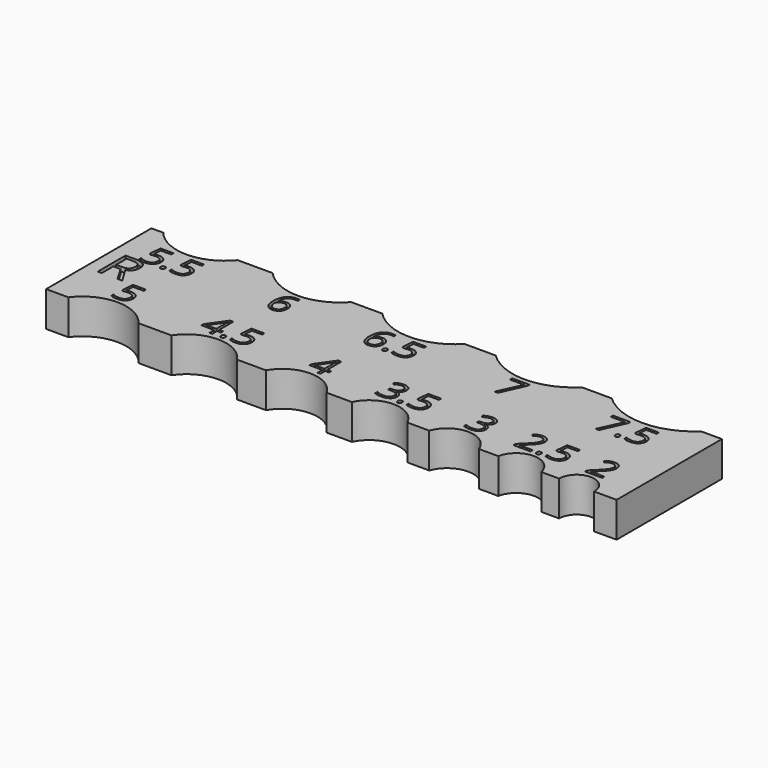
from build123d import *

# Parameters (mm, degrees)
F1_DEPTH       = 4
F2_TEXT_SIZE   = 4.1666666667
F2_TEXT_SIZE_2 = 5.5555555556
F3_DEPTH       = 0.5


# Not quite as in the source:
# - Text() gives the source's letters only with a copy of the font that has no kerning and outlines rounded to 1/6400 em; it was checked with that copy


with BuildPart() as f1:
    # F0 (on Top) → F1 (new body)
    with BuildSketch(Plane.XY):
        with BuildLine():
            Line((-84.5385417342, 32.5298000872), (-84.5385417342, 17.5298000872))
            Line((-84.5385417342, 17.5298000872), (-82.0045393762, 17.5298000872))
            ThreePointArc((-82.0045393762, 17.5298000872), (-78.0045393762, 19.5298000872), (-74.0045393762, 17.5298000872))
            Line((-74.0045393762, 17.5298000872), (-70.2570714699, 17.5298000872))
            ThreePointArc((-70.2570714699, 17.5298000872), (-66.5154140831, 19.5298000872), (-62.7737566964, 17.5298000872))
            Line((-62.7737566964, 17.5298000872), (-59.4914272166, 17.5298000872))
            ThreePointArc((-59.4914272166, 17.5298000872), (-56.0273256014, 19.5298000872), (-52.5632239863, 17.5298000872))
            Line((-52.5632239863, 17.5298000872), (-49.7027702811, 17.5298000872))
            ThreePointArc((-49.7027702811, 17.5298000872), (-46.5404926209, 19.5298000872), (-43.3782149608, 17.5298000872))
            Line((-43.3782149608, 17.5298000872), (-40.8836383714, 17.5298000872))
            ThreePointArc((-40.8836383714, 17.5298000872), (-38.0552112467, 19.5298000872), (-35.226784122, 17.5298000872))
            Line((-35.226784122, 17.5298000872), (-33.0213862159, 17.5298000872))
            ThreePointArc((-33.0213862159, 17.5298000872), (-30.5718964731, 19.5298000872), (-28.1224067304, 17.5298000872))
            Line((-28.1224067304, 17.5298000872), (-26.0911557747, 17.5298000872))
            ThreePointArc((-26.0911557747, 17.5298000872), (-24.0911557747, 19.5298000872), (-22.0911557747, 17.5298000872))
            Line((-22.0911557747, 17.5298000872), (-19.5385417342, 17.5298000872))
            Line((-19.5385417342, 17.5298000872), (-19.5385417342, 32.5298000872))
            Line((-19.5385417342, 32.5298000872), (-21.9044512947, 32.5298000872))
            ThreePointArc((-21.9044512947, 32.5298000872), (-27.0034708083, 30.5298000872), (-32.1024903219, 32.5298000872))
            Line((-32.1024903219, 32.5298000872), (-35.5119116897, 32.5298000872))
            ThreePointArc((-35.5119116897, 32.5298000872), (-40.4108911753, 30.5298000872), (-45.3098706608, 32.5298000872))
            Line((-45.3098706608, 32.5298000872), (-48.8570836346, 32.5298000872))
            ThreePointArc((-48.8570836346, 32.5298000872), (-53.5474993944, 30.5298000872), (-58.2379151542, 32.5298000872))
            Line((-58.2379151542, 32.5298000872), (-61.7753634394, 32.5298000872))
            ThreePointArc((-61.7753634394, 32.5298000872), (-66.2474993944, 30.5298000872), (-70.7196353494, 32.5298000872))
            Line((-70.7196353494, 32.5298000872), (-74.7048587073, 32.5298000872))
            ThreePointArc((-74.7048587073, 32.5298000872), (-78.9474993944, 30.5298000872), (-83.1901400815, 32.5298000872))
            Line((-83.1901400815, 32.5298000872), (-84.5385417342, 32.5298000872))
        make_face()
    extrude(amount=F1_DEPTH)

    # F2 (on face) → F3 (cut)
    with BuildSketch(Plane.XY.offset(4)):
        with Locations((-25.3380647688, 20.0298000872)):
            Text('2', F2_TEXT_SIZE, font='Open Sans', text_align=(TextAlign.LEFT, TextAlign.BOTTOM))
        with Locations((-33.5029522872, 20.0298000872)):
            Text('2.5', F2_TEXT_SIZE, font='Open Sans', text_align=(TextAlign.LEFT, TextAlign.BOTTOM))
        with Locations((-39.2141334956, 20.0298000872)):
            Text('3', F2_TEXT_SIZE, font='Open Sans', text_align=(TextAlign.LEFT, TextAlign.BOTTOM))
        with Locations((-49.3320500397, 20.0298000872)):
            Text('3.5', F2_TEXT_SIZE, font='Open Sans', text_align=(TextAlign.LEFT, TextAlign.BOTTOM))
        with Locations((-57.1463829963, 20.0298000872)):
            Text('4', F2_TEXT_SIZE, font='Open Sans', text_align=(TextAlign.LEFT, TextAlign.BOTTOM))
        with Locations((-69.464603939, 20.0298000872)):
            Text('4.5', F2_TEXT_SIZE, font='Open Sans', text_align=(TextAlign.LEFT, TextAlign.BOTTOM))
        with Locations((-79.4760568305, 20.0298000872)):
            Text('5', F2_TEXT_SIZE, font='Open Sans', text_align=(TextAlign.LEFT, TextAlign.BOTTOM))
        with Locations((-83.6010979135, 23.0298000872)):
            Text('R', F2_TEXT_SIZE_2, font='Open Sans', text_align=(TextAlign.LEFT, TextAlign.BOTTOM))
        with Locations((-81.9381490183, 27.0298000872)):
            Text('5.5', F2_TEXT_SIZE, font='Open Sans', text_align=(TextAlign.LEFT, TextAlign.BOTTOM))
        with Locations((-67.5670455101, 27.0298000872)):
            Text('6', F2_TEXT_SIZE, font='Open Sans', text_align=(TextAlign.LEFT, TextAlign.BOTTOM))
        with Locations((-56.6395822958, 27.0298000872)):
            Text('6.5', F2_TEXT_SIZE, font='Open Sans', text_align=(TextAlign.LEFT, TextAlign.BOTTOM))
        with Locations((-41.6214436107, 27.0298000872)):
            Text('7', F2_TEXT_SIZE, font='Open Sans', text_align=(TextAlign.LEFT, TextAlign.BOTTOM))
        with Locations((-30.1233802604, 27.0298000872)):
            Text('7.5', F2_TEXT_SIZE, font='Open Sans', text_align=(TextAlign.LEFT, TextAlign.BOTTOM))
    extrude(amount=-F3_DEPTH, mode=Mode.SUBTRACT)


solid = f1.part
